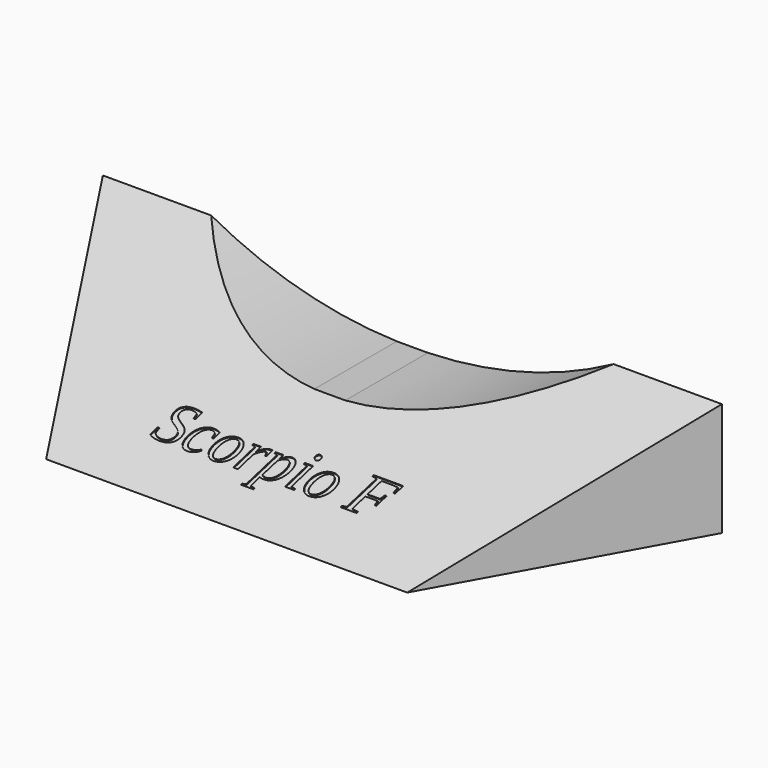
from build123d import *

# Parameters (mm, degrees)
F1_DEPTH      = 110
F3_DEPTH      = 600.001
F4_W          = 30
F4_H          = 100
F5_DEPTH      = 110.001
F7_DEPTH      = 225.001
F8_W          = 30
F8_H          = 61.1111111111
F9_DEPTH      = 100
F10_TEXT_SIZE = 55.5555555556
F11_DEPTH     = 1


# Not quite as in the source:
# - Text() gives the source's letters only with a copy of the font that has no kerning and outlines rounded to 1/6400 em; it was checked with that copy


with BuildPart() as f1:
    # F0 (on Top) → F1 (new body)
    with BuildSketch(Plane.XY):
        Polygon((600, 0), (0, 0), (125, -225), (475, -225), align=None)
    extrude(amount=F1_DEPTH)

    # F2 (on Right) → F3 (cut, through all)
    with BuildSketch(Plane.YZ):
        Polygon((-225, 110), (-225, 0), (0, 110), align=None)
    extrude(amount=F3_DEPTH, mode=Mode.SUBTRACT)

    # F4 (on face) → F5 (cut, through all)
    with BuildSketch(Plane(origin=(0, 0, 0), x_dir=(1, 0, 0), z_dir=(0, 0, -1))):
        with Locations((300, 50)):
            Rectangle(F4_W, F4_H)
    extrude(amount=-F5_DEPTH, mode=Mode.SUBTRACT)

    # F6 (on face) → F7 (cut, through all)
    with BuildSketch(Plane(origin=(0, 0, 0), x_dir=(-1, 0, 0), z_dir=(0, 1, 0))):
        with BuildLine():
            Line((-285, 110), (-285, 61.1111111111))
            ThreePointArc((-285, 61.1111111111), (-192.1105560877, 74.9171484241), (-105, 110))
            Line((-105, 110), (-285, 110))
        make_face()
        with BuildLine():
            Line((-315, 110), (-495, 110))
            ThreePointArc((-495, 110), (-407.8894439123, 74.9171484241), (-315, 61.1111111111))
            Line((-315, 61.1111111111), (-315, 110))
        make_face()
    extrude(amount=-F7_DEPTH, mode=Mode.SUBTRACT)

    # F8 (on face) → F9 (join, through all)
    with BuildSketch(Plane(origin=(0, -100, 0), x_dir=(-1, 0, 0), z_dir=(0, 1, 0))):
        with Locations((-300, 30.5555555556)):
            Rectangle(F8_W, F8_H)
    extrude(amount=F9_DEPTH)

    # F10 (on face) → F11 (cut)
    with BuildSketch(Plane(origin=(0, -43.4037465126, 88.7803905939), x_dir=(1, 0, 0), z_dir=(0, -0.439210132, 0.8983843609))):
        with Locations((187.9079861111, -152.1364812068)):
            Text('Scorpio F', F10_TEXT_SIZE, font='Tinos', font_style=FontStyle.ITALIC, text_align=(TextAlign.LEFT, TextAlign.BOTTOM))
    extrude(amount=-F11_DEPTH, mode=Mode.SUBTRACT)


solid = f1.part
